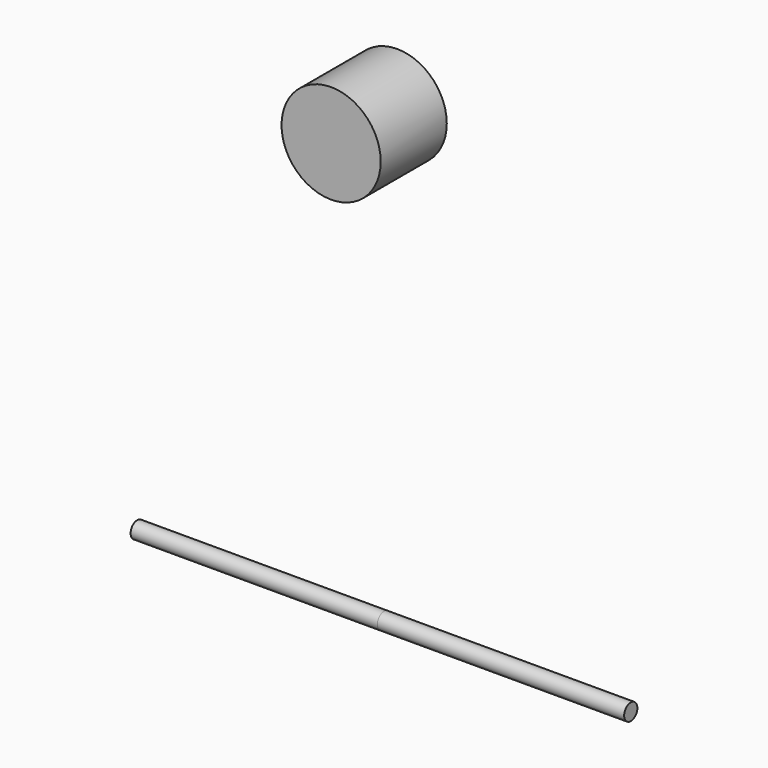
from build123d import *

# Parameters (mm, degrees)
F2_R      = 2.5
F7_R      = 15
F8_DEPTH  = 20
F9_R      = 15
F10_DEPTH = 5


# Not quite as in the source:
# - a pattern or mirror of a feature is missing from the dataset's text; its kind, count and spacing are read off the source's solid


with BuildPart() as f4:
    # F4: sweep along a path in F3
    with BuildLine(Plane.XZ) as f4_path:
        Line((100, 0), (25.3142239141, 0))
    # F2 (on plane+point) → F4 (sweep)
    with BuildSketch(Plane.YZ.offset(100)):
        Circle(F2_R)
    sweep(path=f4_path.line)


with BuildPart() as f4_copies_1:
    # F4_copies: instance of F4
    add(f4.part.mirror(Plane(origin=(100, 0, 0), x_dir=(0, 0, 1), z_dir=(1, 0, 0))))


with BuildPart() as f8:
    # F7 (on Front) → F8 (new body)
    with BuildSketch(Plane.XZ):
        with Locations((100, 135.2881040452)):
            Circle(F7_R)
    extrude(amount=F8_DEPTH)

    # F9 (on face) → F10 (join)
    with BuildSketch(Plane.XZ):
        with Locations((100, 135.2881040452)):
            Circle(F9_R)
    extrude(amount=-F10_DEPTH)


solid = Compound([f4.part, f4_copies_1.part, f8.part])
